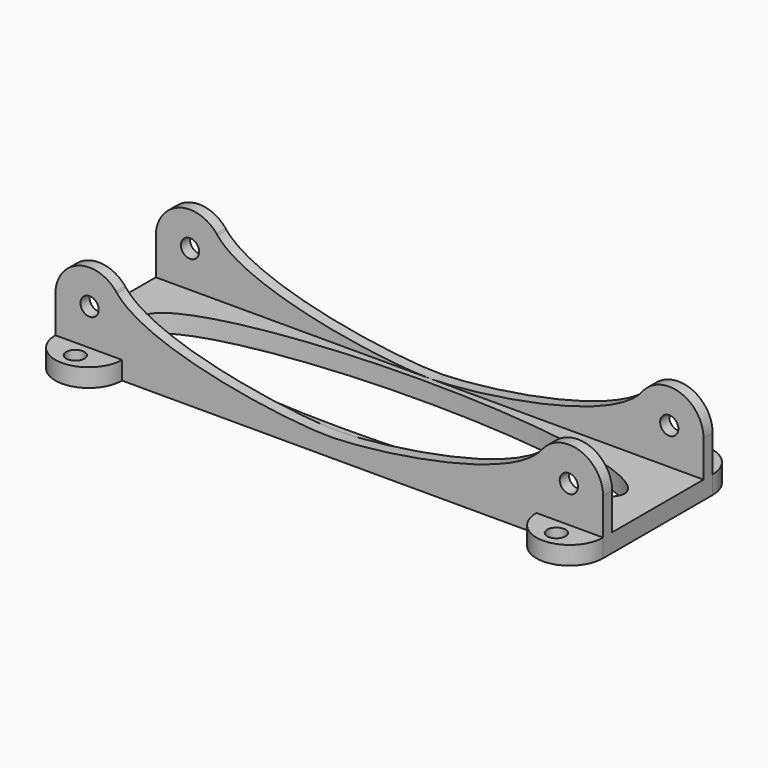
from build123d import *

# Parameters (mm, degrees)
F1_R     = 2
F1_W     = 60
F1_H     = 4
F2_DEPTH = 15
F3_DEPTH = 12.5
F4_R     = 2
F5_DEPTH = 4
F6_DEPTH = 25


with BuildPart() as f2:
    # F1 (on Front) → F2 (new body, symmetric)
    with BuildSketch(Plane.XZ):
        with BuildLine():
            add(Edge.make_bspline(
                [(-46.484745939, 4.4795891086), (-46.5612315065, 4.5731477989), (-46.6348801759, 4.6672380877), (-46.7056330974, 4.7618601615)],
                knots=[47.882184641, 47.882184641, 47.882184641, 47.882184641, 48.4177781173, 48.4177781173, 48.4177781173, 48.4177781173], degree=3))
            ThreePointArc((-46.7056330974, 4.7618601615), (-55.0290559731, 7.0607277164), (-60, 0))
            ThreePointArc((-60, 0), (-52.5, -7.5), (-45, 0))
            ThreePointArc((-45, 0), (-45.3808566015, 2.3596180351), (-46.484745939, 4.4795891086))
        make_face()
        with Locations((-52.5, 0)):
            Circle(F1_R, mode=Mode.SUBTRACT)
        with BuildLine():
            ThreePointArc((-45, 0), (-52.5, -7.5), (-60, 0))
            Line((-60, 0), (-60, -8))
            Line((-60, -8), (0, -8))
            add(Edge.make_bspline(
                [(0, -8), (-10.1354588221, -8), (-39.6469179504, -3.8845801368), (-46.484745939, 4.4795891086)],
                knots=[0, 0, 0, 0, 47.882184641, 47.882184641, 47.882184641, 47.882184641], degree=3))
            ThreePointArc((-46.484745939, 4.4795891086), (-45.3808566015, 2.3596180351), (-45, 0))
        make_face()
        with Locations((-30, -10)):
            Rectangle(F1_W, F1_H)
        with Locations((30, -10)):
            Rectangle(F1_W, F1_H)
        with BuildLine():
            add(Edge.make_bspline(
                [(0, -8), (10.1354588221, -8), (39.6469179504, -3.8845801368), (46.484745939, 4.4795891086)],
                knots=[0, 0, 0, 0, 47.882184641, 47.882184641, 47.882184641, 47.882184641], degree=3))
            Line((0, -8), (60, -8))
            Line((60, -8), (60, 0))
            ThreePointArc((60, 0), (50.1403819649, -7.1191433985), (46.484745939, 4.4795891086))
        make_face()
        with BuildLine():
            add(Edge.make_bspline(
                [(46.484745939, 4.4795891086), (46.5612315065, 4.5731477989), (46.6348801759, 4.6672380877), (46.7056330974, 4.7618601615)],
                knots=[47.882184641, 47.882184641, 47.882184641, 47.882184641, 48.4177781173, 48.4177781173, 48.4177781173, 48.4177781173], degree=3))
            ThreePointArc((46.484745939, 4.4795891086), (50.1403819649, -7.1191433985), (60, 0))
            ThreePointArc((60, 0), (55.0290559731, 7.0607277164), (46.7056330974, 4.7618601615))
        make_face()
        with Locations((52.5, 0)):
            Circle(F1_R, mode=Mode.SUBTRACT)
    extrude(amount=F2_DEPTH, both=True)

    # F1 (on Front) → F3 (cut, symmetric)
    with BuildSketch(Plane.XZ):
        with BuildLine():
            ThreePointArc((-60, 0), (-55.0290559731, 7.0607277164), (-46.7056330974, 4.7618601615))
            ThreePointArc((-46.7056330974, 4.7618601615), (-46.5935030634, 4.6220443461), (-46.484745939, 4.4795891086))
            add(Edge.make_bspline(
                [(0, -8), (-10.1354588221, -8), (-39.6469179504, -3.8845801368), (-46.484745939, 4.4795891086)],
                knots=[0, 0, 0, 0, 47.882184641, 47.882184641, 47.882184641, 47.882184641], degree=3))
            Line((0, -8), (0, 11.9387255982))
            Line((0, 11.9387255982), (-60, 11.9387255982))
            Line((-60, 11.9387255982), (-60, 0))
        make_face()
        with BuildLine():
            Line((0, 11.9387255982), (0, -8))
            add(Edge.make_bspline(
                [(0, -8), (10.1354588221, -8), (39.6469179504, -3.8845801368), (46.484745939, 4.4795891086)],
                knots=[0, 0, 0, 0, 47.882184641, 47.882184641, 47.882184641, 47.882184641], degree=3))
            ThreePointArc((46.484745939, 4.4795891086), (46.5935030634, 4.6220443461), (46.7056330974, 4.7618601615))
            ThreePointArc((46.7056330974, 4.7618601615), (55.0290559731, 7.0607277164), (60, 0))
            Line((60, 0), (60, 11.9387255982))
            Line((60, 11.9387255982), (0, 11.9387255982))
        make_face()
        with BuildLine():
            ThreePointArc((-45, 0), (-52.5, -7.5), (-60, 0))
            Line((-60, 0), (-60, -8))
            Line((-60, -8), (0, -8))
            add(Edge.make_bspline(
                [(0, -8), (-10.1354588221, -8), (-39.6469179504, -3.8845801368), (-46.484745939, 4.4795891086)],
                knots=[0, 0, 0, 0, 47.882184641, 47.882184641, 47.882184641, 47.882184641], degree=3))
            ThreePointArc((-46.484745939, 4.4795891086), (-45.3808566015, 2.3596180351), (-45, 0))
        make_face()
        with BuildLine():
            add(Edge.make_bspline(
                [(0, -8), (10.1354588221, -8), (39.6469179504, -3.8845801368), (46.484745939, 4.4795891086)],
                knots=[0, 0, 0, 0, 47.882184641, 47.882184641, 47.882184641, 47.882184641], degree=3))
            Line((0, -8), (60, -8))
            Line((60, -8), (60, 0))
            ThreePointArc((60, 0), (50.1403819649, -7.1191433985), (46.484745939, 4.4795891086))
        make_face()
        with BuildLine():
            add(Edge.make_bspline(
                [(-46.484745939, 4.4795891086), (-46.5612315065, 4.5731477989), (-46.6348801759, 4.6672380877), (-46.7056330974, 4.7618601615)],
                knots=[47.882184641, 47.882184641, 47.882184641, 47.882184641, 48.4177781173, 48.4177781173, 48.4177781173, 48.4177781173], degree=3))
            ThreePointArc((-46.7056330974, 4.7618601615), (-55.0290559731, 7.0607277164), (-60, 0))
            ThreePointArc((-60, 0), (-52.5, -7.5), (-45, 0))
            ThreePointArc((-45, 0), (-45.3808566015, 2.3596180351), (-46.484745939, 4.4795891086))
        make_face()
        with Locations((-52.5, 0)):
            Circle(F1_R, mode=Mode.SUBTRACT)
        with BuildLine():
            add(Edge.make_bspline(
                [(46.484745939, 4.4795891086), (46.5612315065, 4.5731477989), (46.6348801759, 4.6672380877), (46.7056330974, 4.7618601615)],
                knots=[47.882184641, 47.882184641, 47.882184641, 47.882184641, 48.4177781173, 48.4177781173, 48.4177781173, 48.4177781173], degree=3))
            ThreePointArc((46.484745939, 4.4795891086), (50.1403819649, -7.1191433985), (60, 0))
            ThreePointArc((60, 0), (55.0290559731, 7.0607277164), (46.7056330974, 4.7618601615))
        make_face()
        with Locations((52.5, 0)):
            Circle(F1_R, mode=Mode.SUBTRACT)
        with Locations((-52.5, 0)):
            Circle(F1_R)
        with Locations((52.5, 0)):
            Circle(F1_R)
    extrude(amount=F3_DEPTH, both=True, mode=Mode.SUBTRACT)

    # F4 (on face) → F5 (join)
    with BuildSketch(Plane(origin=(0, 0, -12), x_dir=(1, 0, 0), z_dir=(0, 0, -1))):
        with BuildLine():
            Line((-60, 15), (-45.3916588426, 15))
            ThreePointArc((-45.3916588426, 15), (-52.6958294213, 22.3041705787), (-60, 15))
        make_face()
        with Locations((-52.6958294213, 18.6520852894)):
            Circle(F4_R, mode=Mode.SUBTRACT)
        with BuildLine():
            Line((-45.3916588426, -15), (-60, -15))
            ThreePointArc((-60, -15), (-52.6958294213, -22.3041705787), (-45.3916588426, -15))
        make_face()
        with Locations((-52.6958294213, -18.6520852894)):
            Circle(F4_R, mode=Mode.SUBTRACT)
        with BuildLine():
            ThreePointArc((60, 15), (52.6958294213, 22.3041705787), (45.3916588426, 15))
            Line((45.3916588426, 15), (60, 15))
        make_face()
        with Locations((52.6958294213, 18.6520852894)):
            Circle(F4_R, mode=Mode.SUBTRACT)
        with BuildLine():
            ThreePointArc((45.3916588426, -15), (52.6958294213, -22.3041705787), (60, -15))
            Line((60, -15), (45.3916588426, -15))
        make_face()
        with Locations((52.6958294213, -18.6520852894)):
            Circle(F4_R, mode=Mode.SUBTRACT)
    extrude(amount=-F5_DEPTH)

    # F4 (on face) → F6 (cut)
    with BuildSketch(Plane(origin=(0, 0, -12), x_dir=(1, 0, 0), z_dir=(0, 0, -1))):
        with BuildLine():
            add(Edge.make_bspline(
                [(-52.6958294213, 0), (-52.6958294213, -19.4855715851), (26.3479147106, -9.7427857926), (105.3916588426, 0), (26.3479147106, 9.7427857926), (-52.6958294213, 19.4855715851), (-52.6958294213, 0)],
                knots=[0, 0, 0, 2.0943951024, 2.0943951024, 4.1887902048, 4.1887902048, 6.2831853072, 6.2831853072, 6.2831853072], degree=2, weights=[1, 0.5, 1, 0.5, 1, 0.5, 1]))
        make_face()
    extrude(amount=-F6_DEPTH, mode=Mode.SUBTRACT)


solid = f2.part
